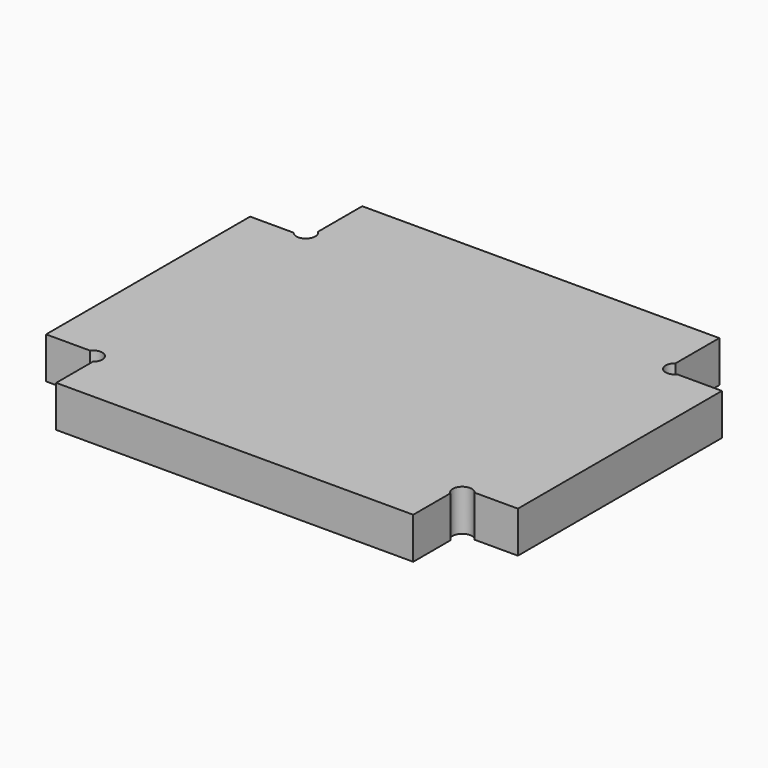
from build123d import *

# Parameters (mm, degrees)
F1_DEPTH = 3.25


# Not quite as in the source:
# - a feature names something its author has since deleted; it is built from what else it names


with BuildPart() as f1:
    # F0 (on Top) → F1 (new body)
    with BuildSketch(Plane.XY):
        with BuildLine():
            Line((-15.0887755982, 9.6346731841), (-18.5, 9.6346731841))
            Line((-18.5, 9.6346731841), (-18.5, -10.3653268159))
            Line((-18.5, -10.3653268159), (-15.0627288748, -10.3653268159))
            ThreePointArc((-15.0627288748, -10.3653268159), (-14.2270313471, -10.1144637876), (-13.719482936, -10.824194178))
            ThreePointArc((-13.719482936, -10.824194178), (-13.7932388225, -11.1485302676), (-14, -11.4090751683))
            Line((-14, -11.4090751683), (-14, -15))
            Line((-14, -15), (14, -15))
            Line((14, -15), (14, -11.3693879251))
            ThreePointArc((14, -11.3693879251), (13.9880219466, -10.2502281458), (15.1013118376, -10.3653268159))
            Line((15.1013118376, -10.3653268159), (18.5, -10.3653268159))
            Line((18.5, -10.3653268159), (18.5, 9.6346731841))
            Line((18.5, 9.6346731841), (15.021365697, 9.6376556492))
            ThreePointArc((15.021365697, 9.6376556492), (13.9052912015, 9.611890406), (14, 10.7242376408))
            Line((14, 10.7242376408), (14, 15))
            Line((14, 15), (-14, 15))
            Line((-14, 15), (-14, 10.6527720123))
            ThreePointArc((-14, 10.6527720123), (-13.8060615496, 10.3964917422), (-13.7372004166, 10.082565248))
            ThreePointArc((-13.7372004166, 10.082565248), (-14.251278169, 9.3706377987), (-15.0887755982, 9.6346731841))
        make_face()
    extrude(amount=F1_DEPTH)


solid = f1.part
